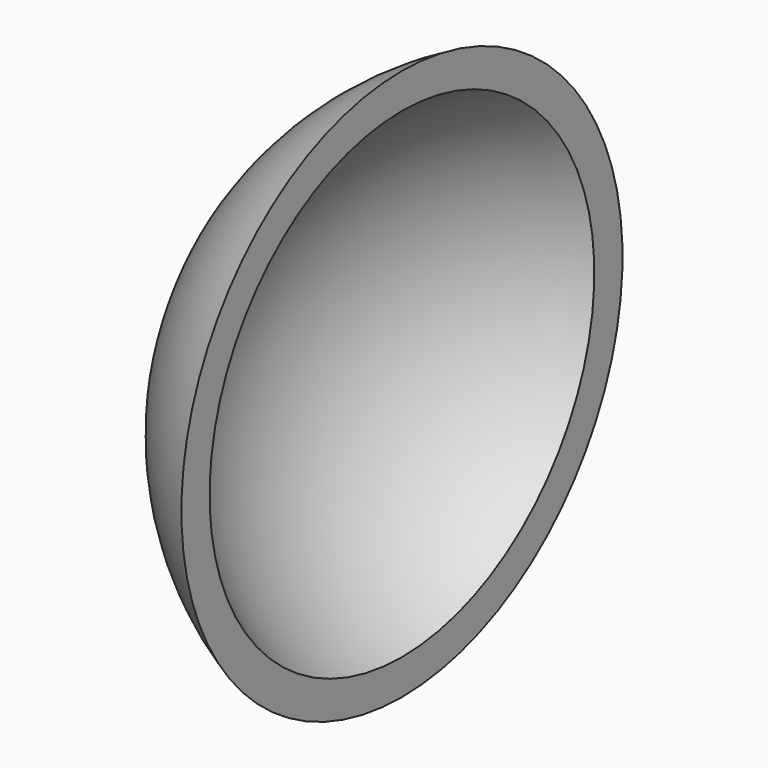
from build123d import *

# Parameters (mm, degrees)
F2_T = -6.35
F3_W = 12.7568915486
F3_H = 15.9924589097


# Not quite as in the source:
# - a feature names something its author has since deleted; it is built from what else it names


with BuildPart() as f1:
    # F0 (on Front) → F1 (revolve)
    with BuildSketch(Plane.XZ):
        with BuildLine():
            Line((39.4908925979, 0), (39.4908925979, 56.4475917369))
            ThreePointArc((39.4908925979, 56.4475917369), (14.1063703184, 33.1501751178), (4.71438, 0))
            Line((4.71438, 0), (39.4908925979, 0))
        make_face()
    revolve(axis=Axis((0, 0, 0), (1, 0, 0)))

    # F2
    f2_openings = [f1.faces().sort_by_distance(p)[0] for p in [
        (39.490893, 0, 0),
    ]]
    offset(amount=F2_T, openings=f2_openings)

    # F3 (on Front) → F4 (revolve, cut)
    with BuildSketch(Plane.XZ):
        with Locations((0, 7.9962294549)):
            Rectangle(F3_W, F3_H)
    revolve(axis=Axis((0, 0, 0), (1, 0, 0)), mode=Mode.SUBTRACT)

    # F5 (on face) → F6 (revolve)
    with BuildSketch(Plane(origin=(6.3784457743, 0, 0), x_dir=(0, -1, 0), z_dir=(-1, 0, 0))):
        Polygon((-1.9871168115, 13.66252359), (0, 0), (0, 13.66252359), align=None)
    revolve(axis=Axis((6.3784457743, 0, 6.831261795), (0, 0, -1)))

    # F5 (on face) → F7 (revolve)
    with BuildSketch(Plane(origin=(6.3784457743, 0, 0), x_dir=(0, -1, 0), z_dir=(-1, 0, 0))):
        Polygon((-8.0306298753, 11.0532137704), (0, 0), (-6.423018605, 12.2212117268), align=None)
    revolve(axis=Axis((6.3784457743, 4.0153149377, 5.5266068852), (0, -0.5877852523, -0.8090169944)))

    # F5 (on face) → F8 (revolve)
    with BuildSketch(Plane(origin=(6.3784457743, 0, 0), x_dir=(0, -1, 0), z_dir=(-1, 0, 0))):
        Polygon((-12.9938320893, 4.2219519754), (0, 0), (-12.3797792248, 6.1118123676), align=None)
    revolve(axis=Axis((6.3784457743, 6.4969160447, 2.1109759877), (0, -0.9510565163, -0.3090169944)))

    # F5 (on face) → F9 (revolve)
    with BuildSketch(Plane(origin=(6.3784457743, 0, 0), x_dir=(0, -1, 0), z_dir=(-1, 0, 0))):
        Polygon((-12.9938320893, -4.2219519754), (0, 0), (-13.6078849539, -2.3320915832), align=None)
    revolve(axis=Axis((6.3784457743, 6.4969160447, -2.1109759877), (0, -0.9510565163, 0.3090169944)))

    # F5 (on face) → F10 (revolve)
    with BuildSketch(Plane(origin=(6.3784457743, 0, 0), x_dir=(0, -1, 0), z_dir=(-1, 0, 0))):
        Polygon((-8.0306298753, -11.0532137704), (0, 0), (-9.6382411456, -9.885215814), align=None)
    revolve(axis=Axis((6.3784457743, 4.0153149377, -5.5266068852), (0, -0.5877852523, 0.8090169944)))

    # F5 (on face) → F11 (revolve)
    with BuildSketch(Plane(origin=(6.3784457743, 0, 0), x_dir=(0, -1, 0), z_dir=(-1, 0, 0))):
        Polygon((0, -13.66252359), (0, 0), (-1.9871168115, -13.66252359), align=None)
    revolve(axis=Axis((6.3784457743, 0, -6.831261795), (0, 0, 1)))

    # F5 (on face) → F12 (revolve)
    with BuildSketch(Plane(origin=(6.3784457743, 0, 0), x_dir=(0, -1, 0), z_dir=(-1, 0, 0))):
        Polygon((6.423018605, 12.2212117268), (0, 0), (8.0306298753, 11.0532137704), align=None)
    revolve(axis=Axis((6.3784457743, -4.0153149377, 5.5266068852), (0, 0.5877852523, -0.8090169944)))

    # F5 (on face) → F13 (revolve)
    with BuildSketch(Plane(origin=(6.3784457743, 0, 0), x_dir=(0, -1, 0), z_dir=(-1, 0, 0))):
        Polygon((12.3797792248, 6.1118123676), (0, 0), (12.9938320893, 4.2219519754), align=None)
    revolve(axis=Axis((6.3784457743, -6.4969160447, 2.1109759877), (0, 0.9510565163, -0.3090169944)))

    # F5 (on face) → F14 (revolve)
    with BuildSketch(Plane(origin=(6.3784457743, 0, 0), x_dir=(0, -1, 0), z_dir=(-1, 0, 0))):
        Polygon((13.6078849539, -2.3320915832), (0, 0), (12.9938320893, -4.2219519754), align=None)
    revolve(axis=Axis((6.3784457743, -6.4969160447, -2.1109759877), (0, 0.9510565163, 0.3090169944)))

    # F5 (on face) → F15 (revolve)
    with BuildSketch(Plane(origin=(6.3784457743, 0, 0), x_dir=(0, -1, 0), z_dir=(-1, 0, 0))):
        Polygon((9.6382411456, -9.885215814), (0, 0), (8.0306298753, -11.0532137704), align=None)
    revolve(axis=Axis((6.3784457743, -4.0153149377, -5.5266068852), (0, 0.5877852523, 0.8090169944)))


solid = f1.part
